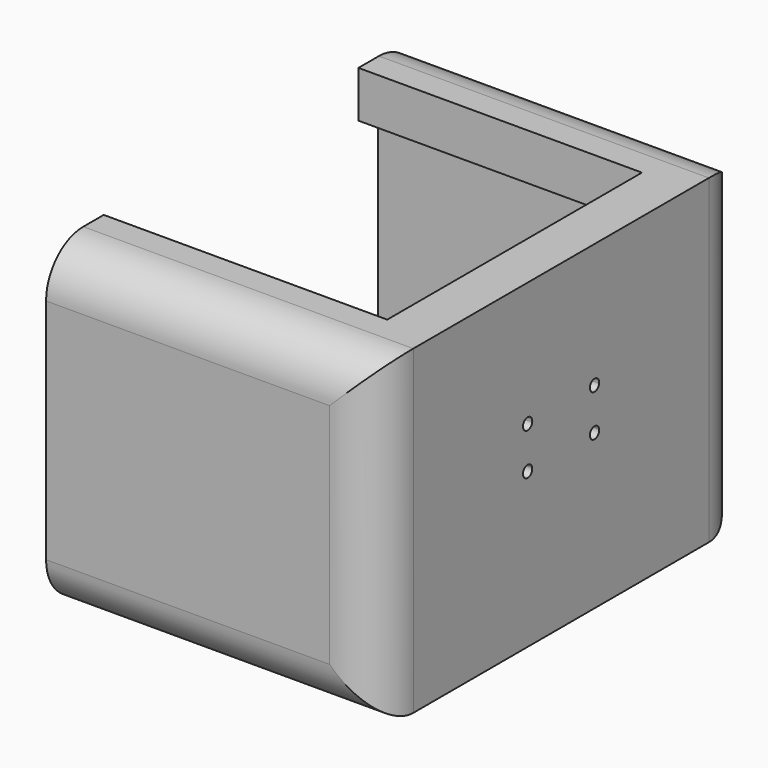
from build123d import *

# Parameters (mm, degrees)
F0_W     = 14.2
F0_H     = 19.9
F1_DEPTH = 13.8
F2_DEPTH = 12
F4_DEPTH = 12.2
F6_DEPTH = 2.001
F7_ANGLE = 180
F8_R     = 2


with BuildPart() as f1:
    # F0 (on Top) → F1 (new body)
    with BuildSketch(Plane.XY):
        with Locations((7.1, 9.95)):
            Rectangle(F0_W, F0_H)
    extrude(amount=F1_DEPTH)

    # F0 (on Top) → F2 (join)
    with BuildSketch(Plane.XY):
        with Locations((7.1, 9.95)):
            Rectangle(F0_W, F0_H)
    extrude(amount=F2_DEPTH)

    # F3 (on face) → F4 (cut)
    with BuildSketch(Plane(origin=(0, 0, 0), x_dir=(0, -1, 0), z_dir=(-1, 0, 0))):
        Polygon((-3.1, 13.8), (-16.8, 13.8), (-16.8, 11.8), (-17.85, 11.8), (-17.85, 2), (-2.05, 2), (-2.05, 11.8), (-3.1, 11.8), align=None)
    extrude(amount=-F4_DEPTH, mode=Mode.SUBTRACT)

    # F5 (on face) → F6 (cut, through all)
    with BuildSketch(Plane(origin=(12.2, 0, 0), x_dir=(0, -1, 0), z_dir=(-1, 0, 0))):
        with BuildLine():
            ThreePointArc((-11.9975769926, 8.4152777778), (-11.75, 8.2), (-11.5024230074, 8.4152777778))
            ThreePointArc((-11.5024230074, 8.4152777778), (-11.75, 8.45), (-11.9975769926, 8.4152777778))
        make_face()
        with BuildLine():
            ThreePointArc((-11.9975769926, 8.4152777778), (-11.75, 8.45), (-11.5024230074, 8.4152777778))
            ThreePointArc((-11.5024230074, 8.4152777778), (-11.5006064875, 8.4325966693), (-11.5, 8.45))
            ThreePointArc((-11.5, 8.45), (-11.7674033307, 8.6993935125), (-11.9975769926, 8.4152777778))
        make_face()
        with BuildLine():
            ThreePointArc((-8.3975769926, 8.4152777778), (-8.15, 8.2), (-7.9024230074, 8.4152777778))
            ThreePointArc((-7.9024230074, 8.4152777778), (-8.15, 8.45), (-8.3975769926, 8.4152777778))
        make_face()
        with BuildLine():
            ThreePointArc((-8.3975769926, 8.4152777778), (-8.15, 8.45), (-7.9024230074, 8.4152777778))
            ThreePointArc((-7.9024230074, 8.4152777778), (-7.9006064875, 8.4325966693), (-7.9, 8.45))
            ThreePointArc((-7.9, 8.45), (-8.1674033307, 8.6993935125), (-8.3975769926, 8.4152777778))
        make_face()
        with BuildLine():
            ThreePointArc((-8.3975769926, 6.6847222222), (-8.15, 6.65), (-7.9024230074, 6.6847222222))
            ThreePointArc((-7.9024230074, 6.6847222222), (-8.15, 6.9), (-8.3975769926, 6.6847222222))
        make_face()
        with BuildLine():
            ThreePointArc((-7.9, 6.65), (-7.9006064875, 6.6674033307), (-7.9024230074, 6.6847222222))
            ThreePointArc((-7.9024230074, 6.6847222222), (-8.15, 6.65), (-8.3975769926, 6.6847222222))
            ThreePointArc((-8.3975769926, 6.6847222222), (-8.1674033307, 6.4006064875), (-7.9, 6.65))
        make_face()
        with BuildLine():
            ThreePointArc((-11.9975769926, 6.6847222222), (-11.75, 6.65), (-11.5024230074, 6.6847222222))
            ThreePointArc((-11.5024230074, 6.6847222222), (-11.75, 6.9), (-11.9975769926, 6.6847222222))
        make_face()
        with BuildLine():
            ThreePointArc((-11.5, 6.65), (-11.5006064875, 6.6674033307), (-11.5024230074, 6.6847222222))
            ThreePointArc((-11.5024230074, 6.6847222222), (-11.75, 6.65), (-11.9975769926, 6.6847222222))
            ThreePointArc((-11.9975769926, 6.6847222222), (-11.7674033307, 6.4006064875), (-11.5, 6.65))
        make_face()
    extrude(amount=-F6_DEPTH, mode=Mode.SUBTRACT)

    # F5 (on face) → F7 (revolve)
    with BuildSketch(Plane(origin=(12.2, 0, 0), x_dir=(0, -1, 0), z_dir=(-1, 0, 0))):
        with BuildLine():
            Line((-12.65, 7.55), (-10.85, 7.55))
            ThreePointArc((-10.85, 7.55), (-11.0313835191, 8.0918397856), (-11.5024230074, 8.4152777778))
            ThreePointArc((-11.5024230074, 8.4152777778), (-11.75, 8.2), (-11.9975769926, 8.4152777778))
            ThreePointArc((-11.9975769926, 8.4152777778), (-12.4686164809, 8.0918397856), (-12.65, 7.55))
        make_face()
        with BuildLine():
            Line((-9.05, 7.55), (-7.25, 7.55))
            ThreePointArc((-7.25, 7.55), (-7.4313835191, 8.0918397856), (-7.9024230074, 8.4152777778))
            ThreePointArc((-7.9024230074, 8.4152777778), (-8.15, 8.2), (-8.3975769926, 8.4152777778))
            ThreePointArc((-8.3975769926, 8.4152777778), (-8.8686164809, 8.0918397856), (-9.05, 7.55))
        make_face()
    revolve(axis=Axis((12.2, 11.75, 7.55), (0, -1, 0)), revolution_arc=F7_ANGLE)

    # F8
    f8_edges = [f1.edges().sort_by_distance(p)[0] for p in [
        (7.1, 0, 0),
        (7.1, 19.9, 0),
        (7.1, 19.9, 13.8),
        (7.1, 0, 13.8),
        (14.2, 0, 6.9),
        (14.2, 19.9, 6.9),
    ]]
    fillet(f8_edges, radius=F8_R)


solid = f1.part
